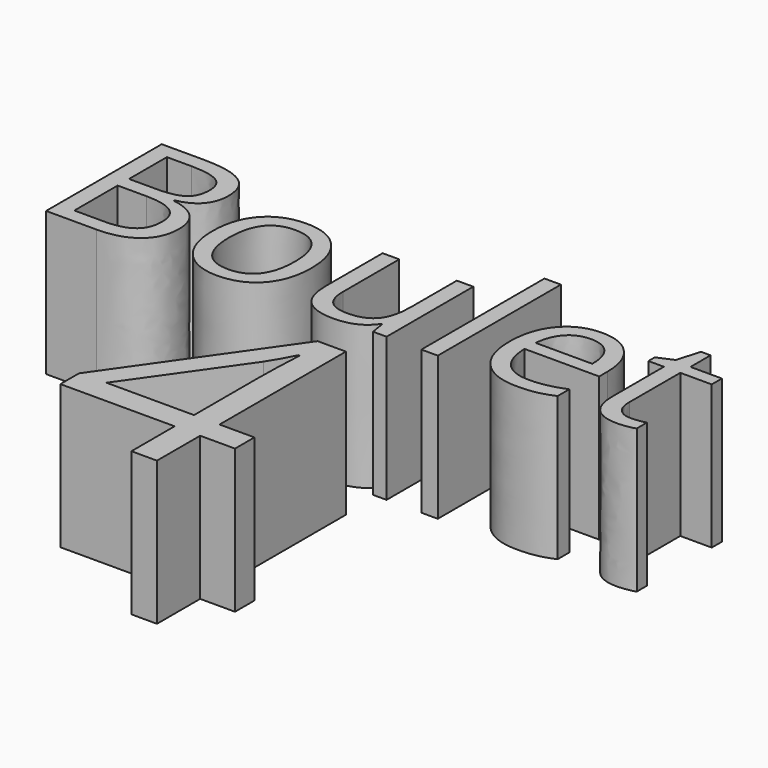
from build123d import *

# Parameters (mm, degrees)
F0_TEXT_SIZE = 8.9496547222
F2_DEPTH     = 6.35
F1_TEXT_SIZE = 14.5431933333
F3_DEPTH     = 6.35


# Not quite as in the source:
# - Text() gives the source's letters only with a copy of the font that has no kerning and outlines rounded to 1/6400 em; it was checked with that copy


with BuildPart() as f2:
    # F0 (on Top) → F2 (new body)
    with BuildSketch(Plane.XY):
        with Locations((-34.6351723391, 26.3503491105)):
            Text('Boulet', F0_TEXT_SIZE, font='Open Sans', text_align=(TextAlign.LEFT, TextAlign.BOTTOM))
    extrude(amount=F2_DEPTH)


with BuildPart() as f3:
    # F1 (on Top) → F3 (new body)
    with BuildSketch(Plane.XY):
        with Locations((-25.5907652136, 14.1652977114)):
            Text('4', F1_TEXT_SIZE, font='Open Sans', text_align=(TextAlign.LEFT, TextAlign.BOTTOM))
    extrude(amount=F3_DEPTH)


solid = Compound([f2.part, f3.part])
